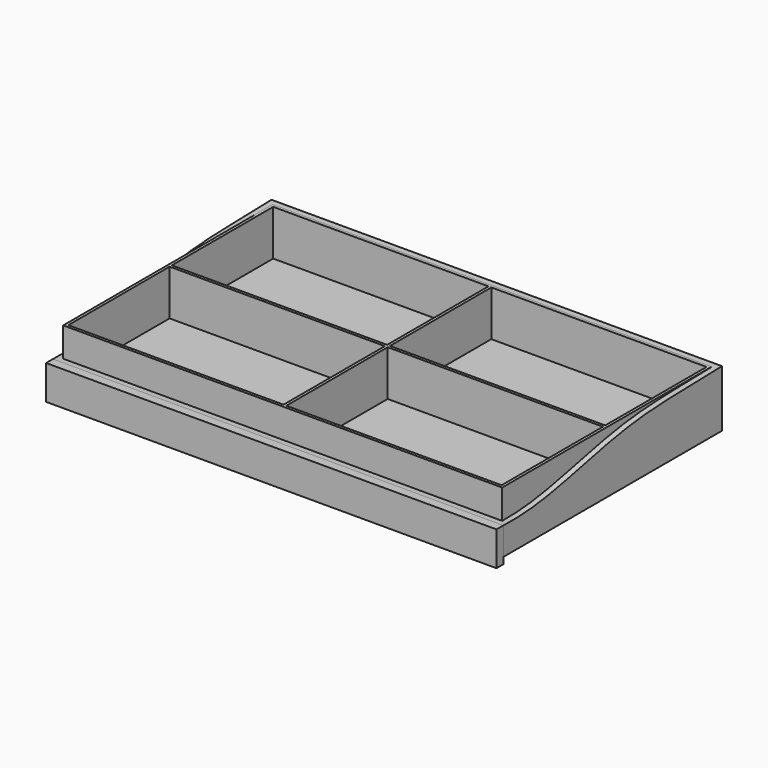
from build123d import *

# Parameters (mm, degrees)
F0_W     = 979.4875
F0_H     = 12.7
F1_DEPTH = 101.6
F2_DEPTH = 25.4
F3_W     = 1004.8875
F3_H     = 609.6
F3_W_2   = 480.21875
F3_H_2   = 282.575
F4_DEPTH = 12.7
F6_DEPTH = 1004.8885
F0_W_2   = 1004.8875
F0_H_2   = 19.05
F7_DEPTH = 36.5125
F8_DEPTH = 39.8145
F0_H_3   = 584.2
F0_W_3   = 480.21875
F0_H_4   = 282.575
F9_DEPTH = 101.6


with BuildPart() as f1:
    # F0 (on Top) → F1 (new body)
    with BuildSketch(Plane.XY):
        Polygon((-74.3194232941, 553.7349042257), (-87.0194232941, 553.7349042257), (-87.0194232941, -55.8650957743), (917.8680767059, -55.8650957743), (917.8680767059, 553.7349042257), (905.1680767059, 553.7349042257), (905.1680767059, 541.0349042257), (905.1680767059, -43.1650957743), (-74.3194232941, -43.1650957743), (-74.3194232941, 541.0349042257), align=None)
        with Locations((415.4243267059, 547.3849042257)):
            Rectangle(F0_W, F0_H)
    extrude(amount=F1_DEPTH)

    # F0 (on Top) → F2 (join)
    with BuildSketch(Plane.XY):
        Polygon((-74.3194232941, 553.7349042257), (-87.0194232941, 553.7349042257), (-87.0194232941, -55.8650957743), (917.8680767059, -55.8650957743), (917.8680767059, 553.7349042257), (905.1680767059, 553.7349042257), (905.1680767059, 541.0349042257), (905.1680767059, -43.1650957743), (-74.3194232941, -43.1650957743), (-74.3194232941, 541.0349042257), align=None)
    extrude(amount=-F2_DEPTH)

    # F3 (on face) → F4 (join)
    with BuildSketch(Plane.XY):
        with Locations((415.4243267059, 248.9349042257)):
            Rectangle(F3_W, F3_H)
        with Locations((658.7087017059, 393.3974042257)):
            Rectangle(F3_W_2, F3_H_2, mode=Mode.SUBTRACT)
        with Locations((658.7087017059, 393.3974042257)):
            Rectangle(F3_W_2, F3_H_2)
    extrude(amount=-F4_DEPTH)

    # F5 (on face) → F6 (cut, through all)
    with BuildSketch(Plane(origin=(-87.0194232941, 0, 0), x_dir=(0, -1, 0), z_dir=(-1, 0, 0))):
        with BuildLine():
            Line((55.8650957743, 101.6), (-553.7349042257, 101.6))
            add(Edge.make_bspline(
                [(-553.7349042257, 101.6), (-479.0590330388, 98.4440573187), (-315.9704193469, 102.4122184163), (-114.0311259776, 50.0416927841), (-5.926719241, 34.1702627815), (55.8650957743, 36.5125)],
                knots=[0, 0, 0, 0, 0.3599583626, 0.6952491461, 1, 1, 1, 1], degree=3))
            Line((55.8650957743, 36.5125), (55.8650957743, 101.6))
        make_face()
    extrude(amount=-F6_DEPTH, mode=Mode.SUBTRACT)


with BuildPart() as f7:
    # F0 (on Top) → F7 (new body)
    with BuildSketch(Plane.XY):
        with Locations((415.4243267059, -65.3900957743)):
            Rectangle(F0_W_2, F0_H_2)
    extrude(amount=F7_DEPTH)

    # F0 (on Top) → F8 (join)
    with BuildSketch(Plane.XY):
        with Locations((415.4243267059, -65.3900957743)):
            Rectangle(F0_W_2, F0_H_2)
    extrude(amount=-F8_DEPTH)


with BuildPart() as f9:
    # F0 (on Top) → F9 (new body)
    with BuildSketch(Plane.XY):
        with Locations((415.4243267059, 248.9349042257)):
            Rectangle(F0_W, F0_H_3)
        with Locations((172.1399517059, 104.4724042257)):
            Rectangle(F0_W_3, F0_H_4, mode=Mode.SUBTRACT)
        with Locations((658.7087017059, 104.4724042257)):
            Rectangle(F0_W_3, F0_H_4, mode=Mode.SUBTRACT)
        with Locations((172.1399517059, 393.3974042257)):
            Rectangle(F0_W_3, F0_H_4, mode=Mode.SUBTRACT)
        with Locations((658.7087017059, 393.3974042257)):
            Rectangle(F0_W_3, F0_H_4, mode=Mode.SUBTRACT)
    extrude(amount=F9_DEPTH)


solid = Compound([f1.part, f7.part, f9.part])
